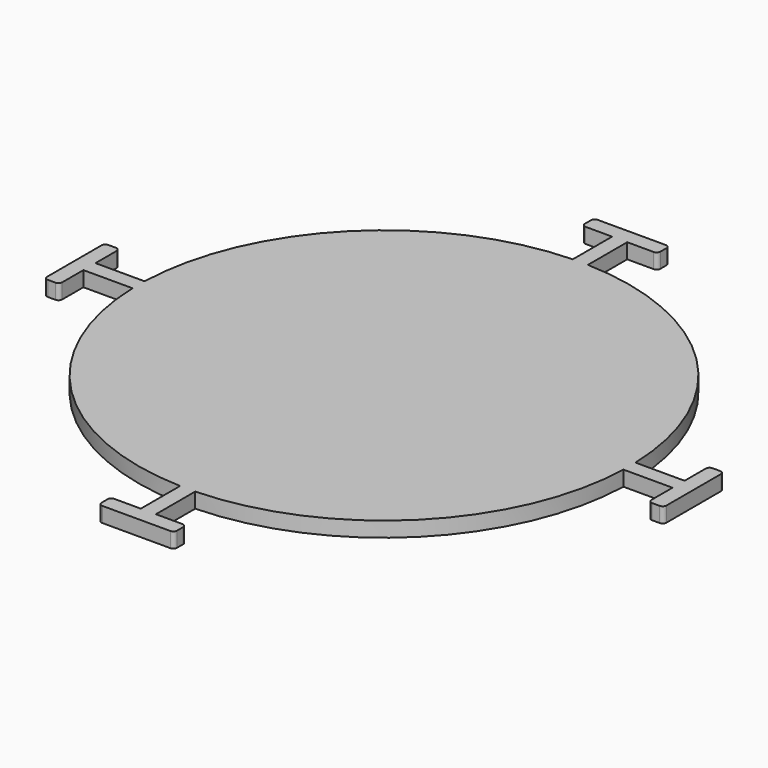
from build123d import *

# Parameters (mm, degrees)
F1_DEPTH = 10.16


with BuildPart() as f1:
    # F0 (on Top) → F1 (new body)
    with BuildSketch(Plane.XY):
        with BuildLine():
            ThreePointArc((165.0218276471, -5.08), (165.080455755, -2.5403007163), (165.1, 0))
            ThreePointArc((165.1, 0), (165.080455755, 2.5403007163), (165.0218276471, 5.08))
            ThreePointArc((165.0218276471, 5.08), (116.7433295739, 116.7433295739), (5.08, 165.0218276471))
            ThreePointArc((5.08, 165.0218276471), (2.5403007163, 165.080455755), (0, 165.1))
            ThreePointArc((0, 165.1), (-2.5403007163, 165.080455755), (-5.08, 165.0218276471))
            ThreePointArc((-5.08, 165.0218276471), (-116.7433295739, 116.7433295739), (-165.0218276471, 5.08))
            ThreePointArc((-165.0218276471, 5.08), (-165.1, 0), (-165.0218276471, -5.08))
            ThreePointArc((-165.0218276471, -5.08), (-116.7433295739, -116.7433295739), (-5.08, -165.0218276471))
            ThreePointArc((-5.08, -165.0218276471), (0, -165.1), (5.08, -165.0218276471))
            ThreePointArc((5.08, -165.0218276471), (116.7433295739, -116.7433295739), (165.0218276471, -5.08))
        make_face()
        with BuildLine():
            ThreePointArc((165.0218276471, 5.08), (165.080455755, 2.5403007163), (165.1, 0))
            ThreePointArc((165.1, 0), (165.080455755, -2.5403007163), (165.0218276471, -5.08))
            Line((165.0218276471, -5.08), (198.0418276471, -5.08))
            Line((198.0418276471, -5.08), (198.0418276471, 5.08))
            Line((198.0418276471, 5.08), (165.0218276471, 5.08))
        make_face()
        with BuildLine():
            ThreePointArc((0, 165.1), (2.5403007163, 165.080455755), (5.08, 165.0218276471))
            Line((5.08, 165.0218276471), (5.08, 198.0418276471))
            Line((5.08, 198.0418276471), (-5.08, 198.0418276471))
            Line((-5.08, 198.0418276471), (-5.08, 165.0218276471))
            ThreePointArc((-5.08, 165.0218276471), (-2.5403007163, 165.080455755), (0, 165.1))
        make_face()
        with BuildLine():
            Line((198.0418276471, 22.86), (198.0418276471, 5.08))
            Line((198.0418276471, 5.08), (203.1218276471, 5.08))
            ThreePointArc((203.1218276471, 5.08), (206.713930094, 3.59210245), (208.2018276471, 4.5e-09))
            Line((208.2018276471, 4.5e-09), (208.2018276471, 22.86))
            ThreePointArc((208.2018276471, 22.86), (207.4578788713, 24.6560512242), (205.6618276471, 25.4))
            Line((205.6618276471, 25.4), (200.5818276471, 25.4))
            ThreePointArc((200.5818276471, 25.4), (198.7857764229, 24.6560512242), (198.0418276471, 22.86))
        make_face()
        with BuildLine():
            Line((203.1218276471, 5.08), (198.0418276471, 5.08))
            Line((198.0418276471, 5.08), (198.0418276471, -5.08))
            Line((198.0418276471, -5.08), (203.1218276471, -5.08))
            ThreePointArc((203.1218276471, -5.08), (206.7139300971, -3.5921024468), (208.2018276471, 4.5e-09))
            ThreePointArc((208.2018276471, 4.5e-09), (206.713930094, 3.59210245), (203.1218276471, 5.08))
        make_face()
        with BuildLine():
            Line((5.08, -198.0418276471), (5.08, -165.0218276471))
            ThreePointArc((5.08, -165.0218276471), (0, -165.1), (-5.08, -165.0218276471))
            Line((-5.08, -165.0218276471), (-5.08, -198.0418276471))
            Line((-5.08, -198.0418276471), (5.08, -198.0418276471))
        make_face()
        with BuildLine():
            Line((203.1218276471, -5.08), (198.0418276471, -5.08))
            Line((198.0418276471, -5.08), (198.0418276471, -22.86))
            ThreePointArc((198.0418276471, -22.86), (198.7857764229, -24.6560512242), (200.5818276471, -25.4))
            Line((200.5818276471, -25.4), (205.6618276471, -25.4))
            ThreePointArc((205.6618276471, -25.4), (207.4578788713, -24.6560512242), (208.2018276471, -22.86))
            Line((208.2018276471, -22.86), (208.2018276471, 4.5e-09))
            ThreePointArc((208.2018276471, 4.5e-09), (206.7139300971, -3.5921024468), (203.1218276471, -5.08))
        make_face()
        with BuildLine():
            Line((-5.08, 198.0418276471), (5.08, 198.0418276471))
            Line((5.08, 198.0418276471), (5.08, 203.1218276471))
            ThreePointArc((5.08, 203.1218276471), (3.5921024559, 206.713930088), (2.13e-08, 208.2018276471))
            ThreePointArc((2.13e-08, 208.2018276471), (-3.5921024409, 206.7139301031), (-5.08, 203.1218276471))
            Line((-5.08, 203.1218276471), (-5.08, 198.0418276471))
        make_face()
        with BuildLine():
            Line((5.08, 203.1218276471), (5.08, 198.0418276471))
            Line((5.08, 198.0418276471), (22.86, 198.0418276471))
            ThreePointArc((22.86, 198.0418276471), (24.6560512242, 198.7857764229), (25.4, 200.5818276471))
            Line((25.4, 200.5818276471), (25.4, 205.6618276471))
            ThreePointArc((25.4, 205.6618276471), (24.6560512242, 207.4578788713), (22.86, 208.2018276471))
            Line((22.86, 208.2018276471), (2.13e-08, 208.2018276471))
            ThreePointArc((2.13e-08, 208.2018276471), (3.5921024559, 206.713930088), (5.08, 203.1218276471))
        make_face()
        with BuildLine():
            Line((22.86, -198.0418276471), (5.08, -198.0418276471))
            Line((5.08, -198.0418276471), (5.08, -203.1218276471))
            ThreePointArc((5.08, -203.1218276471), (3.5921024559, -206.713930088), (2.13e-08, -208.2018276471))
            Line((2.13e-08, -208.2018276471), (22.86, -208.2018276471))
            ThreePointArc((22.86, -208.2018276471), (24.6560512242, -207.4578788713), (25.4, -205.6618276471))
            Line((25.4, -205.6618276471), (25.4, -200.5818276471))
            ThreePointArc((25.4, -200.5818276471), (24.6560512242, -198.7857764229), (22.86, -198.0418276471))
        make_face()
        with BuildLine():
            Line((5.08, -203.1218276471), (5.08, -198.0418276471))
            Line((5.08, -198.0418276471), (-5.08, -198.0418276471))
            Line((-5.08, -198.0418276471), (-5.08, -203.1218276471))
            ThreePointArc((-5.08, -203.1218276471), (-3.5921024409, -206.7139301031), (2.13e-08, -208.2018276471))
            ThreePointArc((2.13e-08, -208.2018276471), (3.5921024559, -206.713930088), (5.08, -203.1218276471))
        make_face()
        with BuildLine():
            Line((-22.86, 198.0418276471), (-5.08, 198.0418276471))
            Line((-5.08, 198.0418276471), (-5.08, 203.1218276471))
            ThreePointArc((-5.08, 203.1218276471), (-3.5921024409, 206.7139301031), (2.13e-08, 208.2018276471))
            Line((2.13e-08, 208.2018276471), (-22.86, 208.2018276471))
            ThreePointArc((-22.86, 208.2018276471), (-24.6560512242, 207.4578788713), (-25.4, 205.6618276471))
            Line((-25.4, 205.6618276471), (-25.4, 200.5818276471))
            ThreePointArc((-25.4, 200.5818276471), (-24.6560512242, 198.7857764229), (-22.86, 198.0418276471))
        make_face()
        with BuildLine():
            Line((-198.0418276471, -5.08), (-165.0218276471, -5.08))
            ThreePointArc((-165.0218276471, -5.08), (-165.1, 0), (-165.0218276471, 5.08))
            Line((-165.0218276471, 5.08), (-198.0418276471, 5.08))
            Line((-198.0418276471, 5.08), (-198.0418276471, -5.08))
        make_face()
        with BuildLine():
            Line((-5.08, -203.1218276471), (-5.08, -198.0418276471))
            Line((-5.08, -198.0418276471), (-22.86, -198.0418276471))
            ThreePointArc((-22.86, -198.0418276471), (-24.6560512242, -198.7857764229), (-25.4, -200.5818276471))
            Line((-25.4, -200.5818276471), (-25.4, -205.6618276471))
            ThreePointArc((-25.4, -205.6618276471), (-24.6560512242, -207.4578788713), (-22.86, -208.2018276471))
            Line((-22.86, -208.2018276471), (2.13e-08, -208.2018276471))
            ThreePointArc((2.13e-08, -208.2018276471), (-3.5921024409, -206.7139301031), (-5.08, -203.1218276471))
        make_face()
        with BuildLine():
            Line((-198.0418276471, -22.86), (-198.0418276471, -5.08))
            Line((-198.0418276471, -5.08), (-203.1218276471, -5.08))
            ThreePointArc((-203.1218276471, -5.08), (-206.7139300971, -3.5921024468), (-208.2018276471, 4.5e-09))
            Line((-208.2018276471, 4.5e-09), (-208.2018276471, -22.86))
            ThreePointArc((-208.2018276471, -22.86), (-207.4578788713, -24.6560512242), (-205.6618276471, -25.4))
            Line((-205.6618276471, -25.4), (-200.5818276471, -25.4))
            ThreePointArc((-200.5818276471, -25.4), (-198.7857764229, -24.6560512242), (-198.0418276471, -22.86))
        make_face()
        with BuildLine():
            Line((-203.1218276471, -5.08), (-198.0418276471, -5.08))
            Line((-198.0418276471, -5.08), (-198.0418276471, 5.08))
            Line((-198.0418276471, 5.08), (-203.1218276471, 5.08))
            ThreePointArc((-203.1218276471, 5.08), (-206.713930094, 3.59210245), (-208.2018276471, 4.5e-09))
            ThreePointArc((-208.2018276471, 4.5e-09), (-206.7139300971, -3.5921024468), (-203.1218276471, -5.08))
        make_face()
        with BuildLine():
            Line((-203.1218276471, 5.08), (-198.0418276471, 5.08))
            Line((-198.0418276471, 5.08), (-198.0418276471, 22.86))
            ThreePointArc((-198.0418276471, 22.86), (-198.7857764229, 24.6560512242), (-200.5818276471, 25.4))
            Line((-200.5818276471, 25.4), (-205.6618276471, 25.4))
            ThreePointArc((-205.6618276471, 25.4), (-207.4578788713, 24.6560512242), (-208.2018276471, 22.86))
            Line((-208.2018276471, 22.86), (-208.2018276471, 4.5e-09))
            ThreePointArc((-208.2018276471, 4.5e-09), (-206.713930094, 3.59210245), (-203.1218276471, 5.08))
        make_face()
    extrude(amount=F1_DEPTH)


solid = f1.part
